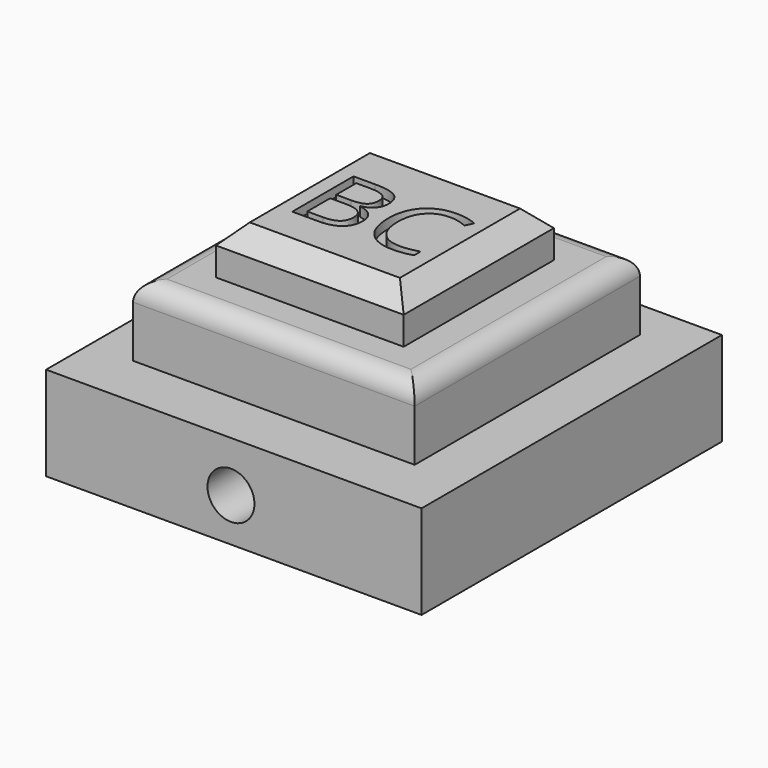
from build123d import *

# Parameters (mm, degrees)
F0_W         = 101.6
F0_H         = 101.6
F1_DEPTH     = 25.4
F2_W         = 76.2
F2_H         = 76.2
F3_DEPTH     = 19.05
F4_W         = 50.8
F4_H         = 50.8
F5_DEPTH     = 12.7
F6_R         = 6.35
F7_DEPTH     = 127
F8_TEXT_SIZE = 28.9975026757
F9_DEPTH     = 2.54
F10_R        = 5.08
F11_SIZE     = 5.08


# Not quite as in the source:
# - Text() gives the source's letters only with a copy of the font that has no kerning and outlines rounded to 1/6400 em; it was checked with that copy


with BuildPart() as f1:
    # F0 (on Top) → F1 (new body)
    with BuildSketch(Plane.XY):
        with Locations((50.8, 50.8)):
            Rectangle(F0_W, F0_H)
    extrude(amount=F1_DEPTH)

    # F2 (on face) → F3 (join)
    with BuildSketch(Plane.XY.offset(25.4)):
        with Locations((49.9255493982, 52.7449047405)):
            Rectangle(F2_W, F2_H)
    extrude(amount=F3_DEPTH)

    # F4 (on face) → F5 (join)
    with BuildSketch(Plane.XY.offset(44.45)):
        with Locations((49.9255871937, 52.1974021259)):
            Rectangle(F4_W, F4_H)
    extrude(amount=F5_DEPTH)

    # F6 (on face) → F7 (cut)
    with BuildSketch(Plane(origin=(0, 101.6, 0), x_dir=(-1, 0, 0), z_dir=(0, 1, 0))):
        with Locations((-50.0326007605, 11.7423580959)):
            Circle(F6_R)
    extrude(amount=-F7_DEPTH, mode=Mode.SUBTRACT)

    # F8 (on face) → F9 (cut)
    with BuildSketch(Plane.XY.offset(57.15)):
        with Locations((30.7206975868, 41.3264889733)):
            Text('BC', F8_TEXT_SIZE, font='Open Sans', text_align=(TextAlign.LEFT, TextAlign.BOTTOM))
    extrude(amount=-F9_DEPTH, mode=Mode.SUBTRACT)

    # F10
    f10_edges = [f1.edges().sort_by_distance(p)[0] for p in [
        (49.925549, 14.644905, 44.45),
        (11.825549, 52.744905, 44.45),
        (88.025549, 52.744905, 44.45),
        (49.925549, 90.844905, 44.45),
    ]]
    fillet(f10_edges, radius=F10_R)

    # F11
    f11_edges = [f1.edges().sort_by_distance(p)[0] for p in [
        (49.925587, 26.797402, 57.15),
        (75.325587, 52.197402, 57.15),
        (49.925587, 77.597402, 57.15),
        (24.525587, 52.197402, 57.15),
    ]]
    chamfer(f11_edges, length=F11_SIZE)


solid = f1.part
